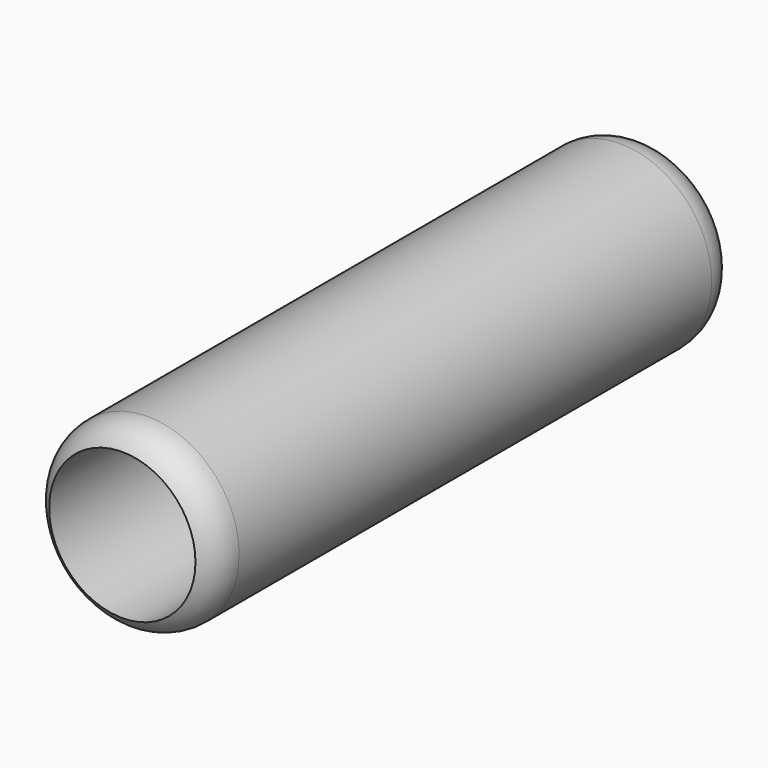
from build123d import *

# Parameters (mm, degrees)
F0_R     = 15.875
F1_DEPTH = 113.5126
F2_R     = 12.7
F3_DEPTH = 113.5126


# Not quite as in the source:
# - a fillet or chamfer that OpenCascade refuses, or shapes differently, is made with other operations: its cross-section is extruded or revolved along the edge and cut away or added


with BuildPart() as f1:
    # F0 (on Front) → F1 (new body)
    with BuildSketch(Plane.XZ):
        Circle(F0_R)
    extrude(amount=F1_DEPTH)

    # F2 (on face) → F3 (cut)
    with BuildSketch(Plane.XZ.offset(113.5126)):
        Circle(F2_R)
    extrude(amount=-F3_DEPTH, mode=Mode.SUBTRACT)

    # F4: fillet of radius 6.35 on 1 edges, made by hand

    # F4_s1 → F4_t2 (revolve, cut)
    with BuildSketch(Plane.XY):
        with BuildLine():
            ThreePointArc((15.875, -108.013338686), (15.024261314, -111.188338686), (12.7, -113.5126))
            Line((12.7, -113.5126), (15.875, -113.5126))
            Line((15.875, -113.5126), (15.875, -108.013338686))
        make_face()
    revolve(axis=Axis((0, -113.5126, 0), (0, -1, 0)), mode=Mode.SUBTRACT)

    # F5: fillet of radius 6.35 on 1 edges, made by hand

    # F5_s1 → F5_t2 (revolve, cut)
    with BuildSketch(Plane.XY):
        with BuildLine():
            ThreePointArc((15.875, -5.499261314), (15.024261314, -2.324261314), (12.7, 0))
            Line((12.7, 0), (15.875, 0))
            Line((15.875, 0), (15.875, -5.499261314))
        make_face()
    revolve(axis=Axis((0, 0, 0), (0, -1, 0)), mode=Mode.SUBTRACT)


solid = f1.part
